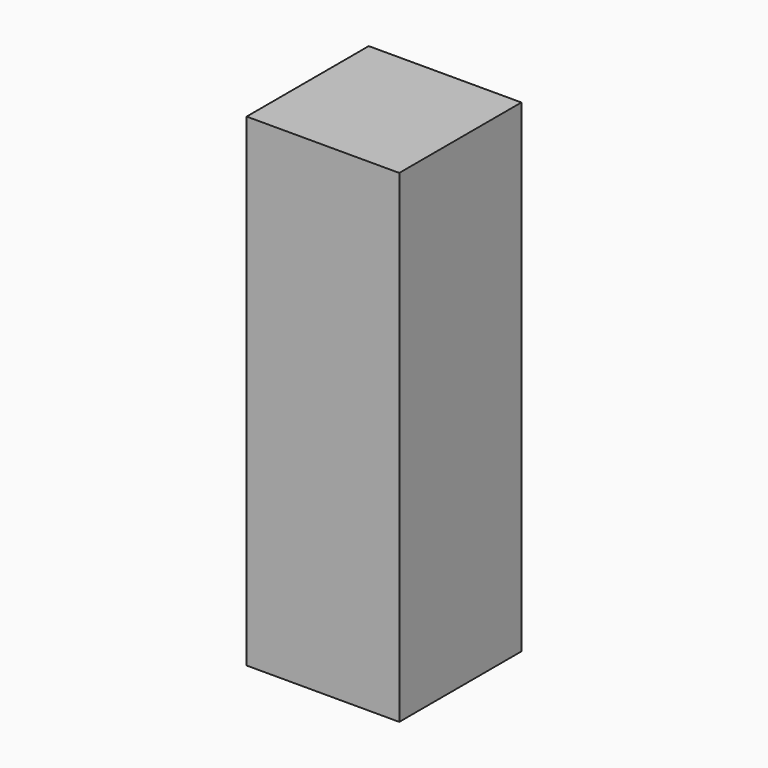
from build123d import *

# Parameters (mm, degrees)
F0_W         = 600
F0_H         = 600
F1_DEPTH     = 1900
F2_TEXT_SIZE = 51.2336691221
F3_DEPTH     = 5


# Not quite as in the source:
# - Text() gives the source's letters only with a copy of the font that has no kerning and outlines rounded to 1/6400 em; it was checked with that copy


with BuildPart() as f1:
    # F0 (on Top) → F1 (new body)
    with BuildSketch(Plane.XY):
        Rectangle(F0_W, F0_H)
    extrude(amount=F1_DEPTH)

    # F2 (on face) → F3 (cut)
    with BuildSketch(Plane(origin=(-300, 0, 0), x_dir=(0, -1, 0), z_dir=(-1, 0, 0))):
        with Locations((-149.1700297532, 1473.8471508026)):
            Text('Fridge', F2_TEXT_SIZE, font='Open Sans', text_align=(TextAlign.LEFT, TextAlign.BOTTOM))
        with Locations((-149.1700297532, 1404.1693607966)):
            Text('Keep', F2_TEXT_SIZE, font='Open Sans', text_align=(TextAlign.LEFT, TextAlign.BOTTOM))
        with Locations((-149.1700297532, 1334.4915707906)):
            Text('Door', F2_TEXT_SIZE, font='Open Sans', text_align=(TextAlign.LEFT, TextAlign.BOTTOM))
        with Locations((-149.1700297532, 1264.8137807846)):
            Text('Clear', F2_TEXT_SIZE, font='Open Sans', text_align=(TextAlign.LEFT, TextAlign.BOTTOM))
    extrude(amount=-F3_DEPTH, mode=Mode.SUBTRACT)


solid = f1.part
